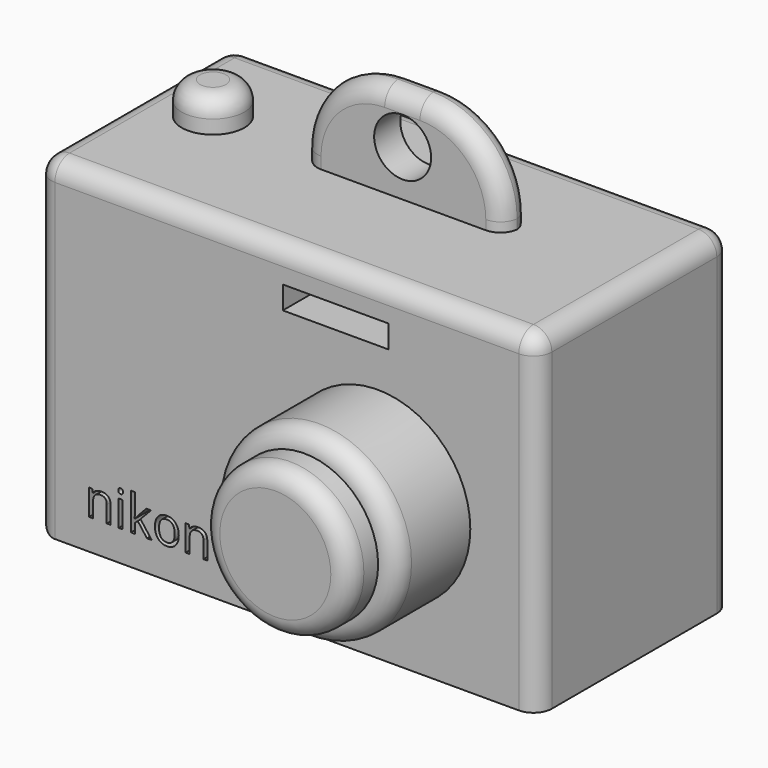
from build123d import *

# Parameters (mm, degrees)
F0_W          = 138.5090965778
F0_H          = 67.2131637111
F1_DEPTH      = 91.948
F2_R          = 25.6222846106
F3_DEPTH      = 25.4
F4_R          = 20.4340282328
F5_DEPTH      = 10
F6_R          = 5.08
F7_R          = 5.08
F8_R          = 8.6707638381
F9_DEPTH      = 8.89
F11_W         = 29.2187072337
F11_H         = 6.3221603632
F10_TEXT_SIZE = 13.4017434902
F12_DEPTH     = 25.4
F13_DEPTH     = 25.4
F14_DEPTH     = 25.4
F15_TEXT_SIZE = 16.2400926153
F16_DEPTH     = 25.4
F17_W         = 104.1087135673
F17_H         = 56.8241644651
F18_DEPTH     = 2.794
F19_W         = 55.7491630316
F19_H         = 9.0460889041
F20_DEPTH     = 25.908
F21_R         = 22.6887790592
F22_R         = 23.301989304
F23_R         = 7.8822987347
F24_DEPTH     = 45.974
F25_T3_ANGLE  = 90
F25_T6_ANGLE  = 90
F25_T9_DEPTH  = 3.2192209408
F25_T12_DEPTH = 9.7583946684
F25_T15_ANGLE = 90
F25_T18_DEPTH = 2.606010696
F25_T21_DEPTH = 3.2192209408
F25_T24_DEPTH = 9.7583946684
F25_T27_ANGLE = 90
F25_T30_DEPTH = 2.606010696
F26_R         = 5.08


# Not quite as in the source:
# - a fillet or chamfer that OpenCascade refuses, or shapes differently, is made with other operations: its cross-section is extruded or revolved along the edge and cut away or added
# - Text() gives the source's letters only with a copy of the font that has no kerning and outlines rounded to 1/6400 em; it was checked with that copy


with BuildPart() as f1:
    # F0 (on Top) → F1 (new body)
    with BuildSketch(Plane.XY):
        with Locations((-48.4346142039, -23.8942014985)):
            Rectangle(F0_W, F0_H)
    extrude(amount=F1_DEPTH)

    # F2 (on face) → F3 (join)
    with BuildSketch(Plane.XZ.offset(57.500783354)):
        with Locations((-23.2952851802, 39.8159623146)):
            Circle(F2_R)
    extrude(amount=F3_DEPTH)

    # F4 (on face) → F5 (join)
    with BuildSketch(Plane.XZ.offset(82.900783354)):
        with Locations((-23.2952851802, 39.8159623146)):
            Circle(F4_R)
    extrude(amount=F5_DEPTH)

    # F6
    f6_edges = [f1.edges().sort_by_distance(p)[0] for p in [
        (-43.729313, -92.900783, 39.815962),
        (20.819934, -23.894201, 91.948),
        (-117.689162, -23.894201, 91.948),
        (-48.91757, -82.900783, 39.815962),
    ]]
    fillet(f6_edges, radius=F6_R)

    # F7
    f7_edges = [f1.edges().sort_by_distance(p)[0] for p in [
        (-117.689162, 9.71238, 43.434),
        (-117.689162, -23.894201, 86.868),
        (-117.689162, -23.894201, 0),
        (-117.689162, -57.500783, 43.434),
    ]]
    fillet(f7_edges, radius=F7_R)

    # F8 (on face) → F9 (join)
    with BuildSketch(Plane.XY.offset(91.948)):
        with Locations((-99.2026105523, -19.5780303329)):
            Circle(F8_R)
    extrude(amount=F9_DEPTH)

    # F11 (on face) + F10 (on face) → F12 (cut)
    with BuildSketch(Plane.XZ.offset(57.500783354)):
        with Locations((-34.9331777543, 79.3584659696)):
            Rectangle(F11_W, F11_H)
    with BuildSketch(Plane.XZ.offset(57.500783354)):
        with Locations((-104.3271124363, 8.462597616)):
            Text('nikon', F10_TEXT_SIZE, font='Open Sans', text_align=(TextAlign.LEFT, TextAlign.BOTTOM))
    extrude(amount=-F12_DEPTH, mode=Mode.SUBTRACT)

    # F13 (cut): a face of the model
    f13_faces = [f1.faces().sort_by_distance(p)[0] for p in [
        (-34.9331777543, -32.100783354, 79.3584659696),
    ]]
    extrude(f13_faces, amount=-F13_DEPTH, mode=Mode.SUBTRACT)

    # F14 (cut): a face of the model
    f14_faces = [f1.faces().sort_by_distance(p)[0] for p in [
        (-34.9331777543, -6.700783354, 79.3584659696),
    ]]
    extrude(f14_faces, amount=-F14_DEPTH, mode=Mode.SUBTRACT)

    # F15 (on face) → F16 (cut)
    with BuildSketch(Plane(origin=(0, 9.7123803571, 0), x_dir=(-1, 0, 0), z_dir=(0, 1, 0))):
        with Locations((-11.8789179251, 70.968195796)):
            Text('hd', F15_TEXT_SIZE, font='Open Sans', text_align=(TextAlign.LEFT, TextAlign.BOTTOM))
    extrude(amount=-F16_DEPTH, mode=Mode.SUBTRACT)

    # F17 (on face) → F18 (cut)
    with BuildSketch(Plane(origin=(0, 9.7123803571, 0), x_dir=(-1, 0, 0), z_dir=(0, 1, 0))):
        with Locations((52.0543567836, 36.2159823999)):
            Rectangle(F17_W, F17_H)
    extrude(amount=-F18_DEPTH, mode=Mode.SUBTRACT)

    # F19 (on face) → F20 (join)
    with BuildSketch(Plane.XY.offset(91.948)):
        with Locations((-42.6234975457, -19.9209712446)):
            Rectangle(F19_W, F19_H)
    extrude(amount=F20_DEPTH)

    # F21
    f21_edges = [f1.edges().sort_by_distance(p)[0] for p in [
        (-70.498079, -19.920971, 117.856),
    ]]
    fillet(f21_edges, radius=F21_R)

    # F22
    f22_edges = [f1.edges().sort_by_distance(p)[0] for p in [
        (-14.748916, -19.920971, 117.856),
    ]]
    fillet(f22_edges, radius=F22_R)

    # F23 (on face) → F24 (cut)
    with BuildSketch(Plane.XZ.offset(24.4440156966)):
        with Locations((-42.834546417, 104.7215908766)):
            Circle(F23_R)
    extrude(amount=-F24_DEPTH, mode=Mode.SUBTRACT)

    # F25: fillet of radius 5.08 on 2 edges, made by hand


with BuildPart() as f25_tool1:
    # F25_s2 → F25_t3 (revolve)
    with BuildSketch(Plane.XY.offset(95.1672209408)):
        with BuildLine():
            ThreePointArc((-70.4980790615, -19.3640156966), (-69.0101815099, -22.9561181451), (-65.4180790615, -24.4440156966))
            Line((-65.4180790615, -24.4440156966), (-65.4180790615, -24.5456156966))
            Line((-65.4180790615, -24.5456156966), (-70.5996790615, -24.5456156966))
            Line((-70.5996790615, -24.5456156966), (-70.5996790615, -19.3640156966))
            Line((-70.5996790615, -19.3640156966), (-70.4980790615, -19.3640156966))
        make_face()
    revolve(axis=Axis((-47.8093000023, -24.4440156966, 95.1672209408), (0, 1, 0)), revolution_arc=F25_T3_ANGLE)


with BuildPart() as f25_tool4:
    # F25_s5 → F25_t6 (revolve)
    with BuildSketch(Plane.XY.offset(95.1672209408)):
        with BuildLine():
            ThreePointArc((-65.4180790615, -15.3979267925), (-69.0101815099, -16.8858243441), (-70.4980790615, -20.4779267925))
            Line((-70.4980790615, -20.4779267925), (-70.5996790615, -20.4779267925))
            Line((-70.5996790615, -20.4779267925), (-70.5996790615, -15.2963267925))
            Line((-70.5996790615, -15.2963267925), (-65.4180790615, -15.2963267925))
            Line((-65.4180790615, -15.2963267925), (-65.4180790615, -15.3979267925))
        make_face()
    revolve(axis=Axis((-47.8093000023, -15.3979267925, 95.1672209408), (0, 1, 0)), revolution_arc=F25_T6_ANGLE)


with BuildPart() as f25_tool7:
    # F25_s8 → F25_t9 (new body)
    with BuildSketch(Plane.XY.offset(91.948)):
        with BuildLine():
            ThreePointArc((-65.4180790615, -15.3979267925), (-69.0101815099, -16.8858243441), (-70.4980790615, -20.4779267925))
            Line((-70.4980790615, -20.4779267925), (-70.5996790615, -20.4779267925))
            Line((-70.5996790615, -20.4779267925), (-70.5996790615, -15.2963267925))
            Line((-70.5996790615, -15.2963267925), (-65.4180790615, -15.2963267925))
            Line((-65.4180790615, -15.2963267925), (-65.4180790615, -15.3979267925))
        make_face()
    extrude(amount=F25_T9_DEPTH)


with BuildPart() as f25_tool10:
    # F25_s11 → F25_t12 (new body)
    with BuildSketch(Plane.YZ.offset(-38.050905334)):
        with BuildLine():
            ThreePointArc((-15.3979267925, 112.776), (-16.8858243441, 116.3681024484), (-20.4779267925, 117.856))
            Line((-20.4779267925, 117.856), (-20.4779267925, 117.9576))
            Line((-20.4779267925, 117.9576), (-15.2963267925, 117.9576))
            Line((-15.2963267925, 117.9576), (-15.2963267925, 112.776))
            Line((-15.2963267925, 112.776), (-15.3979267925, 112.776))
        make_face()
    extrude(amount=-F25_T12_DEPTH)


with BuildPart() as f25_tool13:
    # F25_s14 → F25_t15 (revolve)
    with BuildSketch(Plane.YZ.offset(-38.050905334)):
        with BuildLine():
            ThreePointArc((-15.3979267925, 112.776), (-16.8858243441, 116.3681024484), (-20.4779267925, 117.856))
            Line((-20.4779267925, 117.856), (-20.4779267925, 117.9576))
            Line((-20.4779267925, 117.9576), (-15.2963267925, 117.9576))
            Line((-15.2963267925, 117.9576), (-15.2963267925, 112.776))
            Line((-15.2963267925, 112.776), (-15.3979267925, 112.776))
        make_face()
    revolve(axis=Axis((-38.050905334, -15.3979267925, 94.554010696), (0, 1, 0)), revolution_arc=F25_T15_ANGLE)


with BuildPart() as f25_tool16:
    # F25_s17 → F25_t18 (new body)
    with BuildSketch(Plane.XY.offset(91.948)):
        with BuildLine():
            ThreePointArc((-19.8289160299, -15.3979267925), (-16.2368135815, -16.8858243441), (-14.7489160299, -20.4779267925))
            Line((-14.7489160299, -20.4779267925), (-14.6473160299, -20.4779267925))
            Line((-14.6473160299, -20.4779267925), (-14.6473160299, -15.2963267925))
            Line((-14.6473160299, -15.2963267925), (-19.8289160299, -15.2963267925))
            Line((-19.8289160299, -15.2963267925), (-19.8289160299, -15.3979267925))
        make_face()
    extrude(amount=F25_T18_DEPTH)


with BuildPart() as f25_tool19:
    # F25_s20 → F25_t21 (new body)
    with BuildSketch(Plane.XY.offset(91.948)):
        with BuildLine():
            ThreePointArc((-70.4980790615, -19.3640156966), (-69.0101815099, -22.9561181451), (-65.4180790615, -24.4440156966))
            Line((-65.4180790615, -24.4440156966), (-65.4180790615, -24.5456156966))
            Line((-65.4180790615, -24.5456156966), (-70.5996790615, -24.5456156966))
            Line((-70.5996790615, -24.5456156966), (-70.5996790615, -19.3640156966))
            Line((-70.5996790615, -19.3640156966), (-70.4980790615, -19.3640156966))
        make_face()
    extrude(amount=F25_T21_DEPTH)


with BuildPart() as f25_tool22:
    # F25_s23 → F25_t24 (new body)
    with BuildSketch(Plane.YZ.offset(-47.8093000023)):
        with BuildLine():
            ThreePointArc((-19.3640156966, 117.856), (-22.9561181451, 116.3681024484), (-24.4440156966, 112.776))
            Line((-24.4440156966, 112.776), (-24.5456156966, 112.776))
            Line((-24.5456156966, 112.776), (-24.5456156966, 117.9576))
            Line((-24.5456156966, 117.9576), (-19.3640156966, 117.9576))
            Line((-19.3640156966, 117.9576), (-19.3640156966, 117.856))
        make_face()
    extrude(amount=F25_T24_DEPTH)


with BuildPart() as f25_tool25:
    # F25_s26 → F25_t27 (revolve)
    with BuildSketch(Plane.YZ.offset(-38.050905334)):
        with BuildLine():
            ThreePointArc((-19.3640156966, 117.856), (-22.9561181451, 116.3681024484), (-24.4440156966, 112.776))
            Line((-24.4440156966, 112.776), (-24.5456156966, 112.776))
            Line((-24.5456156966, 112.776), (-24.5456156966, 117.9576))
            Line((-24.5456156966, 117.9576), (-19.3640156966, 117.9576))
            Line((-19.3640156966, 117.9576), (-19.3640156966, 117.856))
        make_face()
    revolve(axis=Axis((-38.050905334, -24.4440156966, 94.554010696), (0, 1, 0)), revolution_arc=F25_T27_ANGLE)


with BuildPart() as f25_tool28:
    # F25_s29 → F25_t30 (new body)
    with BuildSketch(Plane.XY.offset(91.948)):
        with BuildLine():
            ThreePointArc((-14.7489160299, -19.3640156966), (-16.2368135815, -22.9561181451), (-19.8289160299, -24.4440156966))
            Line((-19.8289160299, -24.4440156966), (-19.8289160299, -24.5456156966))
            Line((-19.8289160299, -24.5456156966), (-14.6473160299, -24.5456156966))
            Line((-14.6473160299, -24.5456156966), (-14.6473160299, -19.3640156966))
            Line((-14.6473160299, -19.3640156966), (-14.7489160299, -19.3640156966))
        make_face()
    extrude(amount=F25_T30_DEPTH)


with BuildPart() as f1_1:
    add(f1.part)

    # F25_t31: cut F25_tool1, F25_tool4, F25_tool7, F25_tool10, F25_tool13, F25_tool16, F25_tool19, F25_tool22, F25_tool25, F25_tool28
    add([f25_tool1.part, f25_tool4.part, f25_tool7.part, f25_tool10.part, f25_tool13.part, f25_tool16.part, f25_tool19.part, f25_tool22.part, f25_tool25.part, f25_tool28.part], mode=Mode.SUBTRACT)

    # F26
    f26_edges = [f1_1.edges().sort_by_distance(p)[0] for p in [
        (-107.873374, -19.57803, 100.838),
    ]]
    fillet(f26_edges, radius=F26_R)


solid = f1_1.part
